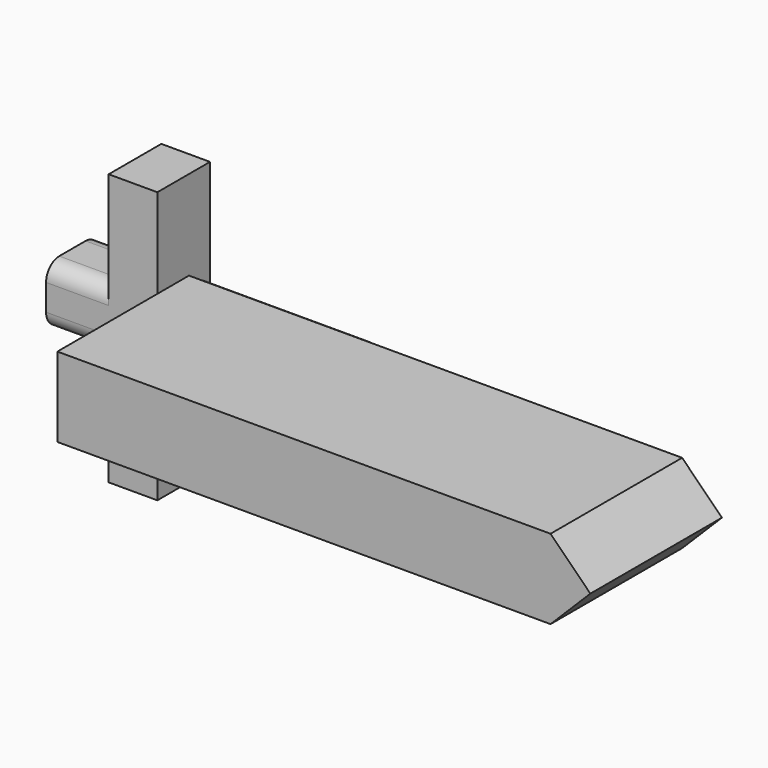
from build123d import *

# Parameters (mm, degrees)
F0_W        = 25.5065411329
F0_H        = 9.1286599636
F0_W_2      = 9.6656344831
F0_W_3      = 7.5177252293
F0_H_2      = 15.3039256111
F0_H_3      = 17.4518460408
F1_DEPTH    = 5.08
F2_R        = 2.54
F3_R        = 2.54
F4_W        = 86.313597858
F4_H        = 12.2866295278
F5_DEPTH    = 25.4
F6_T1_DEPTH = 77.6565983155


# Not quite as in the source:
# - a fillet or chamfer that OpenCascade refuses, or shapes differently, is made with other operations: its cross-section is extruded or revolved along the edge and cut away or added


with BuildPart() as f1:
    # F0 (on Front) → F1 (new body, symmetric)
    with BuildSketch(Plane.XZ):
        with Locations((-64.7060722113, 33.9639782906)):
            Rectangle(F0_W, F0_H)
        with Locations((-89.8098852485, 33.9639782906)):
            Rectangle(F0_W_2, F0_H)
        with Locations((-81.2182053924, 46.1802710779)):
            Rectangle(F0_W_3, F0_H_2)
        with Locations((-81.2182053924, 33.9639782906)):
            Rectangle(F0_W_3, F0_H)
        with Locations((-81.2182053924, 20.6737252884)):
            Rectangle(F0_W_3, F0_H_3)
    extrude(amount=F1_DEPTH, both=True)

    # F2
    f2_edges = [f1.edges().sort_by_distance(p)[0] for p in [
        (-64.706072, -5.08, 38.528308),
        (-89.809885, -5.08, 38.528308),
    ]]
    fillet(f2_edges, radius=F2_R)

    # F3
    f3_edges = [f1.edges().sort_by_distance(p)[0] for p in [
        (-64.706072, -5.08, 29.399648),
        (-89.809885, -5.08, 29.399648),
        (-89.809885, 5.08, 29.399648),
        (-64.706072, 5.08, 29.399648),
        (-64.706072, 5.08, 38.528308),
        (-89.809885, 5.08, 38.528308),
    ]]
    fillet(f3_edges, radius=F3_R)

    # F4 (on Front) → F5 (join)
    with BuildSketch(Plane.XZ):
        with Locations((-33.4874503314, 34.556152299)):
            Rectangle(F4_W, F4_H)
    extrude(amount=F5_DEPTH)

    # F6: chamfer of 10.16 on 2 edges, made by hand

    # F6_s2 → F6_t1 (cut)
    with BuildSketch(Plane.XZ.offset(-26.1282991577)):
        Polygon((-0.4906514025, 40.699467063), (9.6693485975, 30.539467063), (9.6693485975, 40.699467063), align=None)
        Polygon((9.6693485975, 38.5728375351), (-0.4906514025, 28.4128375351), (9.6693485975, 28.4128375351), align=None)
    extrude(amount=F6_T1_DEPTH, mode=Mode.SUBTRACT)


solid = f1.part
